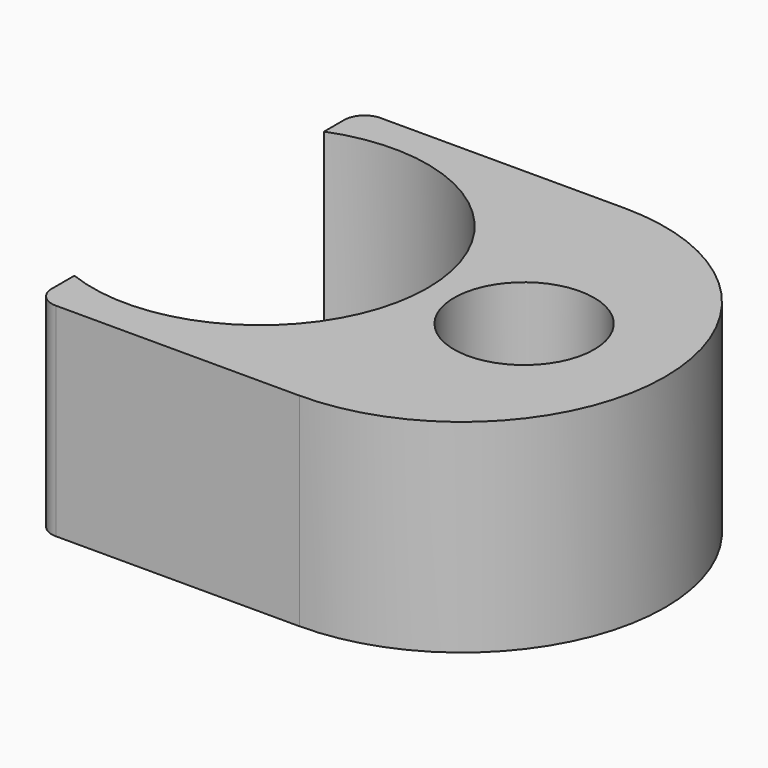
from build123d import *

# Parameters (mm, degrees)
F0_R     = 6.9
F1_DEPTH = 20
F3_R     = 2


# Not quite as in the source:
# - a feature of the source that left no trace in its solid (it failed there, or was rolled back) is left out


with BuildPart() as f1:
    # F0 (on Top) → F1 (new body)
    with BuildSketch(Plane.XY):
        with BuildLine():
            ThreePointArc((-6, 15.3704261489), (9.3072552345, 13.6244265934), (16.5, 0))
            ThreePointArc((16.5, 0), (9.3072552345, -13.6244265934), (-6, -15.3704261489))
            Line((-6, -15.3704261489), (-6, -20.1503510079))
            Line((-6, -20.1503510079), (-6, -20.1573419994))
            Line((-6, -20.1573419994), (19.9984760751, -20.1573419994))
            ThreePointArc((19.9984760751, -20.1573419994), (40.0019715709, -0.1538465036), (19.9984760751, 19.8496489921))
            Line((19.9984760751, 19.8496489921), (-6, 19.8496489921))
            Line((-6, 19.8496489921), (-6, 15.3704261489))
        make_face()
        with Locations((26, 0)):
            Circle(F0_R, mode=Mode.SUBTRACT)
    extrude(amount=F1_DEPTH)

    # F3
    f3_edges = [f1.edges().sort_by_distance(p)[0] for p in [
        (-6, -20.157342, 10),
        (-6, 19.849649, 10),
    ]]
    fillet(f3_edges, radius=F3_R)


solid = f1.part
